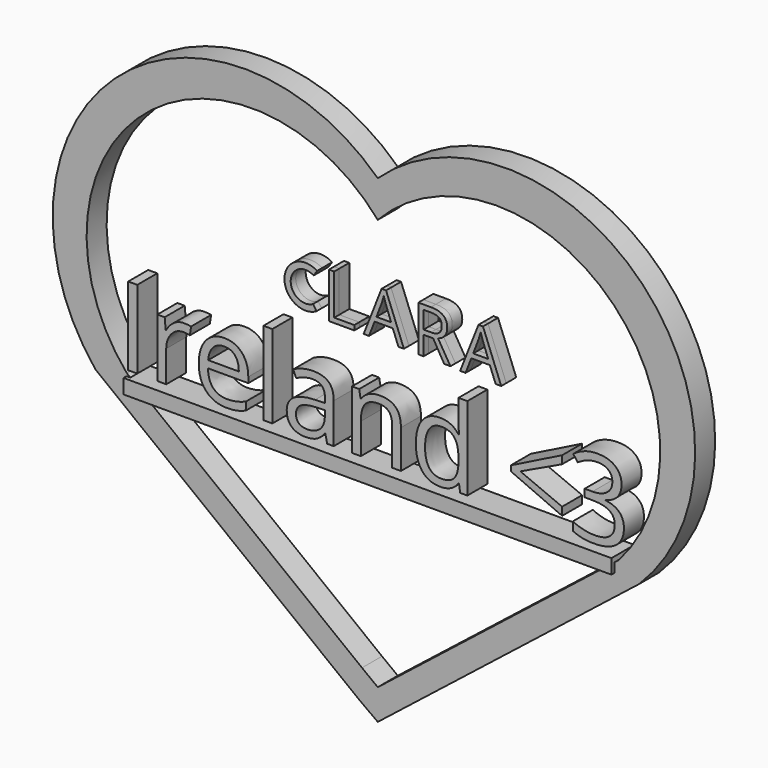
from build123d import *

# Parameters (mm, degrees)
F0_TEXT_SIZE   = 129.7821523622
F0_TEXT_SIZE_2 = 131.8390481174
F0_TEXT_SIZE_3 = 129.1353669431
F0_TEXT_SIZE_4 = 129.1688816208
F1_DEPTH       = 25.4
F2_DEPTH       = 12.7
F3_TEXT_SIZE   = 222.2182953523
F4_DEPTH       = 50.8
F5_W           = 990.8061027527
F5_H           = 14.7751867771
F6_DEPTH       = 58.42
F9_DEPTH       = 50.8


# Not quite as in the source:
# - Text() gives the source's letters only with a copy of the font that has no kerning and outlines rounded to 1/6400 em; it was checked with that copy


with BuildPart() as f1:
    # F0 (on Front) → F1 (new body)
    with BuildSketch(Plane.XZ):
        with BuildLine():
            Line((-140.4435635898, 43.0940349789), (-133.4106167681, 53.6695142963))
            ThreePointArc((-133.4106167681, 53.6695142963), (-199.6771450614, 18.4001099995), (-134.3711418546, -18.6175830221))
            Line((-134.3711418546, -18.6175830221), (-141.6711095171, -8.188130639))
            ThreePointArc((-141.6711095171, -8.188130639), (-186.9722981731, 18.5520228402), (-140.4435635898, 43.0940349789))
        make_face()
        with Locations((59.4596378505, -28.6848153919)):
            Text('R', F0_TEXT_SIZE, font='Open Sans', text_align=(TextAlign.LEFT, TextAlign.BOTTOM))
        with Locations((157.1156829596, -30.5746421218)):
            Text('A', F0_TEXT_SIZE_2, font='Open Sans', text_align=(TextAlign.LEFT, TextAlign.BOTTOM))
        with Locations((-38.8042218983, -28.2191298902)):
            Text('A', F0_TEXT_SIZE_3, font='Open Sans', text_align=(TextAlign.LEFT, TextAlign.BOTTOM))
        with Locations((-121.9274625182, -28.2432604581)):
            Text('L', F0_TEXT_SIZE_4, font='Open Sans', text_align=(TextAlign.LEFT, TextAlign.BOTTOM))
    extrude(amount=F1_DEPTH)


with BuildPart() as f2:
    # F2 (new): a face of the model
    f2_faces = [f1.part.faces().sort_by_distance(p)[0] for p in [
        (-138.9083430038, -25.4, -14.0238537433),
    ]]
    extrude(f2_faces, amount=F2_DEPTH)


with BuildPart() as f2b:
    # F2#2 (new): a face of the model
    f2_2_faces = [f1.part.faces().sort_by_distance(p)[0] for p in [
        (-99.5915316001, -25.4, 22.7178998688),
    ]]
    extrude(f2_2_faces, amount=F2_DEPTH)


with BuildPart() as f2c:
    # F2#3 (new): a face of the model
    f2_3_faces = [f1.part.faces().sort_by_distance(p)[0] for p in [
        (27.2260130178, -25.4, -13.1099815306),
    ]]
    extrude(f2_3_faces, amount=F2_DEPTH)


with BuildPart() as f2d:
    # F2#4 (new): a face of the model
    f2_4_faces = [f1.part.faces().sort_by_distance(p)[0] for p in [
        (81.8289967685, -25.4, -9.4202771506),
    ]]
    extrude(f2_4_faces, amount=F2_DEPTH)


with BuildPart() as f2e:
    # F2#5 (new): a face of the model
    f2_5_faces = [f1.part.faces().sort_by_distance(p)[0] for p in [
        (224.5283796078, -25.4, -15.1491565654),
    ]]
    extrude(f2_5_faces, amount=F2_DEPTH)


with BuildPart() as f4:
    # F3 (on Front) → F4 (new body)
    with BuildSketch(Plane.XZ):
        with Locations((-528.6402208731, -240.1957288384)):
            Text('Ireland <3', F3_TEXT_SIZE, font='Open Sans', text_align=(TextAlign.LEFT, TextAlign.BOTTOM))
    extrude(amount=F4_DEPTH)


with BuildPart() as f6:
    # F5 (on Front) → F6 (new body)
    with BuildSketch(Plane.XZ):
        with Locations((-14.8359835148, -259.2958658934)):
            Rectangle(F5_W, F5_H)
        with Locations((-14.8359835148, -274.0710526705)):
            Rectangle(F5_W, F5_H)
    extrude(amount=F6_DEPTH)

    # F8 (on face) → F9 (join)
    with BuildSketch(Plane.XZ):
        with BuildLine():
            Line((-573.5391704375, -260.1223631995), (-38.8294421136, -675.8898496628))
            Line((-38.8294421136, -675.8898496628), (0, -704.0719389915))
            Line((0, -704.0719389915), (530.6809918161, -285.0291625925))
            ThreePointArc((530.6809918161, -285.0291625925), (537.8549701346, 252.9859082749), (0, 267.9429650307))
            ThreePointArc((0, 267.9429650307), (-534.046056545, 272.4807497812), (-573.5391704375, -260.1223631995))
        make_face()
        with BuildLine():
            ThreePointArc((0, 193.4414369166), (466.0366891627, 210.1260644398), (489.3163412531, -255.6277656463))
            Line((489.3163412531, -255.6277656463), (0, -642.0076837859))
            Line((0, -642.0076837859), (-31.9992564619, -617.747426033))
            Line((-31.9992564619, -617.747426033), (-509.4926953316, -246.4688867331))
            ThreePointArc((-509.4926953316, -246.4688867331), (-474.7015094906, 228.2326227576), (0, 193.4414369166))
        make_face(mode=Mode.SUBTRACT)
    extrude(amount=F9_DEPTH)


solid = Compound([f1.part, f2.part, f2b.part, f2c.part, f2d.part, f2e.part, f4.part, f6.part])
